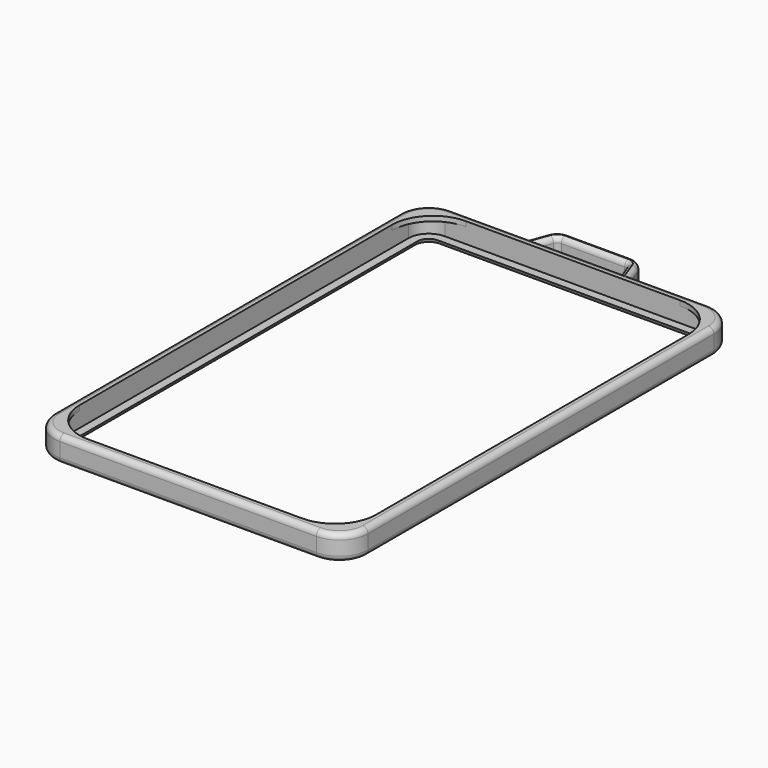
from build123d import *

# Parameters (mm, degrees)
F2_DEPTH      = 2.8
F4_DEPTH      = 0.9
F6_DEPTH      = 0.9
F8_DEPTH      = 3.7
F8_DEPTH_BACK = 0.9
F9_T1_DEPTH   = 79.28
F9_T3_DEPTH   = 11.5995849236
F9_T5_DEPTH   = 47.03
F9_T10_DEPTH  = 4.9923257792
F9_T15_DEPTH  = 20.1838214056
F9_T20_DEPTH  = 20.1838214056
F9_T26_DEPTH  = 20.1838214056
F9_T31_DEPTH  = 20.1838214056
F9_T36_DEPTH  = 20.1838214056
F9_T42_DEPTH  = 20.1838214056
F9_T45_ANGLE  = 90
F9_T47_ANGLE  = 90
F9_T49_ANGLE  = 90
F9_T51_ANGLE  = 90
F9_T53_ANGLE  = 90
F9_T57_DEPTH  = 16.7204048612
F9_T62_DEPTH  = 16.7204048612
F9_T67_DEPTH  = 16.7204048612
F9_T72_DEPTH  = 16.7204048612
F9_T75_ANGLE  = 90
F9_T77_ANGLE  = 90
F9_T81_DEPTH  = 16.7204048612
F9_T86_DEPTH  = 16.7204048612
F9_T91_DEPTH  = 16.7204048612
F9_T96_DEPTH  = 16.7204048612
F9_T99_ANGLE  = 90
F9_T101_ANGLE = 90
F9_T103_ANGLE = 90
F9_T105_ANGLE = 90
F9_T107_ANGLE = 90
F9_T109_ANGLE = 70
F9_T111_ANGLE = 70
F9_T115_DEPTH = 4.9923257792
F9_T120_DEPTH = 4.9923257792
F9_T123_ANGLE = 70
F9_T125_ANGLE = 70
F9_T129_DEPTH = 5.574678154
F9_T134_DEPTH = 5.574678154
F9_T137_ANGLE = 70
F9_T139_ANGLE = 70
F9_T143_DEPTH = 5.574678154
F9_T148_DEPTH = 5.574678154
F9_T151_ANGLE = 70
F9_T153_ANGLE = 70
F9_T157_DEPTH = 4.9923257792
F9_T163_DEPTH = 20.1838214056
F9_T168_DEPTH = 4.9923257792
F9_T175_DEPTH = 20.1838214056
F9_T180_DEPTH = 4.9923257792
F9_T187_DEPTH = 20.1838214056
F9_T192_DEPTH = 4.9923257792
F9_T199_DEPTH = 20.1838214056
F9_T204_DEPTH = 4.9923257792
F9_T211_DEPTH = 16.7204048612
F9_T216_DEPTH = 5.574678154
F9_T223_DEPTH = 5.574678154
F9_T227_DEPTH = 16.7204048612
F9_T235_DEPTH = 16.7204048612
F9_T240_DEPTH = 5.574678154
F9_T247_DEPTH = 5.574678154
F9_T251_DEPTH = 16.7204048612


# Not quite as in the source:
# - a fillet or chamfer that OpenCascade refuses, or shapes differently, is made with other operations: its cross-section is extruded or revolved along the edge and cut away or added


with BuildPart() as f2:
    # F1 (on Top) → F2 (new body)
    with BuildSketch(Plane.XY):
        with BuildLine():
            Line((-28.8, 39.64), (-28.8, -39.64))
            ThreePointArc((-28.8, -39.64), (-27.2520593386, -43.3770593386), (-23.515, -44.925))
            Line((-23.515, -44.925), (23.515, -44.925))
            ThreePointArc((23.515, -44.925), (27.2520593386, -43.3770593386), (28.8, -39.64))
            Line((28.8, -39.64), (28.8, 39.64))
            ThreePointArc((28.8, 39.64), (27.2520593386, 43.3770593386), (23.515, 44.925))
            Line((23.515, 44.925), (-23.515, 44.925))
            ThreePointArc((-23.515, 44.925), (-27.2520593386, 43.3770593386), (-28.8, 39.64))
        make_face()
        with BuildLine():
            ThreePointArc((-23.515, -43.325), (-26.1206884887, -42.2456884887), (-27.2, -39.64))
            Line((-27.2, -39.64), (-27.2, 39.64))
            ThreePointArc((-27.2, 39.64), (-26.1206884887, 42.2456884887), (-23.515, 43.325))
            Line((-23.515, 43.325), (23.515, 43.325))
            ThreePointArc((23.515, 43.325), (26.1206884887, 42.2456884887), (27.2, 39.64))
            Line((27.2, 39.64), (27.2, -39.64))
            ThreePointArc((27.2, -39.64), (26.1206884887, -42.2456884887), (23.515, -43.325))
            Line((23.515, -43.325), (-23.515, -43.325))
        make_face(mode=Mode.SUBTRACT)
    extrude(amount=F2_DEPTH)

    # F3 (on face) → F4 (join)
    with BuildSketch(Plane(origin=(0, 0, 0), x_dir=(1, 0, 0), z_dir=(0, 0, -1))):
        with BuildLine():
            Line((28.8, -39.64), (28.8, 39.64))
            ThreePointArc((28.8, 39.64), (27.2520593386, 43.3770593386), (23.515, 44.925))
            Line((23.515, 44.925), (-23.515, 44.925))
            ThreePointArc((-23.515, 44.925), (-27.2520593386, 43.3770593386), (-28.8, 39.64))
            Line((-28.8, 39.64), (-28.8, -39.64))
            ThreePointArc((-28.8, -39.64), (-27.2520593386, -43.3770593386), (-23.515, -44.925))
            Line((-23.515, -44.925), (23.515, -44.925))
            ThreePointArc((23.515, -44.925), (27.2520593386, -43.3770593386), (28.8, -39.64))
        make_face()
        with BuildLine():
            Line((-23.515, 43.325), (23.515, 43.325))
            ThreePointArc((23.515, 43.325), (26.1206884887, 42.2456884887), (27.2, 39.64))
            Line((27.2, 39.64), (27.2, -39.64))
            ThreePointArc((27.2, -39.64), (26.1206884887, -42.2456884887), (23.515, -43.325))
            Line((23.515, -43.325), (-23.515, -43.325))
            ThreePointArc((-23.515, -43.325), (-26.1206884887, -42.2456884887), (-27.2, -39.64))
            Line((-27.2, -39.64), (-27.2, 39.64))
            ThreePointArc((-27.2, 39.64), (-26.1206884887, 42.2456884887), (-23.515, 43.325))
        make_face(mode=Mode.SUBTRACT)
        with BuildLine():
            ThreePointArc((27.2, 39.64), (26.1206884887, 42.2456884887), (23.515, 43.325))
            Line((23.515, 43.325), (-23.515, 43.325))
            ThreePointArc((-23.515, 43.325), (-26.1206884887, 42.2456884887), (-27.2, 39.64))
            Line((-27.2, 39.64), (-27.2, -39.64))
            ThreePointArc((-27.2, -39.64), (-26.1206884887, -42.2456884887), (-23.515, -43.325))
            Line((-23.515, -43.325), (23.515, -43.325))
            ThreePointArc((23.515, -43.325), (26.1206884887, -42.2456884887), (27.2, -39.64))
            Line((27.2, -39.64), (27.2, 39.64))
        make_face()
        with BuildLine():
            Line((-25.6, -39.64), (-25.6, 39.64))
            ThreePointArc((-25.6, 39.64), (-24.9893176388, 41.1143176388), (-23.515, 41.725))
            Line((-23.515, 41.725), (23.515, 41.725))
            ThreePointArc((23.515, 41.725), (24.9893176388, 41.1143176388), (25.6, 39.64))
            Line((25.6, 39.64), (25.6, -39.64))
            ThreePointArc((25.6, -39.64), (24.9893176388, -41.1143176388), (23.515, -41.725))
            Line((23.515, -41.725), (-23.515, -41.725))
            ThreePointArc((-23.515, -41.725), (-24.9893176388, -41.1143176388), (-25.6, -39.64))
        make_face(mode=Mode.SUBTRACT)
    extrude(amount=F4_DEPTH)

    # F5 (on face) → F6 (join)
    with BuildSketch(Plane.XY.offset(2.8)):
        with BuildLine():
            Line((-23.515, -44.925), (23.515, -44.925))
            ThreePointArc((23.515, -44.925), (27.2520593386, -43.3770593386), (28.8, -39.64))
            Line((28.8, -39.64), (28.8, 39.64))
            ThreePointArc((28.8, 39.64), (27.2520593386, 43.3770593386), (23.515, 44.925))
            Line((23.515, 44.925), (-23.515, 44.925))
            ThreePointArc((-23.515, 44.925), (-27.2520593386, 43.3770593386), (-28.8, 39.64))
            Line((-28.8, 39.64), (-28.8, -39.64))
            ThreePointArc((-28.8, -39.64), (-27.2520593386, -43.3770593386), (-23.515, -44.925))
        make_face()
        with BuildLine():
            Line((19.6522583002, 43.325), (23.515, 43.325))
            ThreePointArc((23.515, 43.325), (26.1206884887, 42.2456884887), (27.2, 39.64))
            Line((27.2, 39.64), (27.2, 35.7772583002))
            Line((27.2, 35.7772583002), (27.2, -35.7772583002))
            Line((27.2, -35.7772583002), (27.2, -39.64))
            ThreePointArc((27.2, -39.64), (26.1206884887, -42.2456884887), (23.515, -43.325))
            Line((23.515, -43.325), (19.6522583002, -43.325))
            Line((19.6522583002, -43.325), (-19.6522583002, -43.325))
            Line((-19.6522583002, -43.325), (-23.515, -43.325))
            ThreePointArc((-23.515, -43.325), (-26.1206884887, -42.2456884887), (-27.2, -39.64))
            Line((-27.2, -39.64), (-27.2, -35.7772583002))
            Line((-27.2, -35.7772583002), (-27.2, 35.7772583002))
            Line((-27.2, 35.7772583002), (-27.2, 39.64))
            ThreePointArc((-27.2, 39.64), (-26.1206884887, 42.2456884887), (-23.515, 43.325))
            Line((-23.515, 43.325), (-19.6522583002, 43.325))
            Line((-19.6522583002, 43.325), (19.6522583002, 43.325))
        make_face(mode=Mode.SUBTRACT)
        with BuildLine():
            ThreePointArc((-27.2, 35.7772583002), (-24.9893176388, 41.1143176388), (-19.6522583002, 43.325))
            Line((-19.6522583002, 43.325), (-23.515, 43.325))
            ThreePointArc((-23.515, 43.325), (-26.1206884887, 42.2456884887), (-27.2, 39.64))
            Line((-27.2, 39.64), (-27.2, 35.7772583002))
        make_face()
        with BuildLine():
            ThreePointArc((27.2, 39.64), (26.1206884887, 42.2456884887), (23.515, 43.325))
            Line((23.515, 43.325), (19.6522583002, 43.325))
            ThreePointArc((19.6522583002, 43.325), (24.9893176388, 41.1143176388), (27.2, 35.7772583002))
            Line((27.2, 35.7772583002), (27.2, 39.64))
        make_face()
        with BuildLine():
            Line((27.2, -39.64), (27.2, -35.7772583002))
            ThreePointArc((27.2, -35.7772583002), (24.9893176388, -41.1143176388), (19.6522583002, -43.325))
            Line((19.6522583002, -43.325), (23.515, -43.325))
            ThreePointArc((23.515, -43.325), (26.1206884887, -42.2456884887), (27.2, -39.64))
        make_face()
        with BuildLine():
            ThreePointArc((-19.6522583002, -43.325), (-24.9893176388, -41.1143176388), (-27.2, -35.7772583002))
            Line((-27.2, -35.7772583002), (-27.2, -39.64))
            ThreePointArc((-27.2, -39.64), (-26.1206884887, -42.2456884887), (-23.515, -43.325))
            Line((-23.515, -43.325), (-19.6522583002, -43.325))
        make_face()
    extrude(amount=F6_DEPTH)

    # F7 (on Top) → F8 (join, two sides)
    with BuildSketch(Plane.XY) as f8_sk:
        with BuildLine():
            Line((-9.2945951388, 44.925), (-7.5919107028, 44.925))
            Line((-7.5919107028, 44.925), (-6.7394850826, 47.2670201433))
            ThreePointArc((-6.7394850826, 47.2670201433), (-6.3733688981, 47.7441520443), (-5.7997924618, 47.925))
            Line((-5.7997924618, 47.925), (5.7997924618, 47.925))
            ThreePointArc((5.7997924618, 47.925), (6.3733688981, 47.7441520443), (6.7394850826, 47.2670201433))
            Line((6.7394850826, 47.2670201433), (7.5919107028, 44.925))
            Line((7.5919107028, 44.925), (9.2945951388, 44.925))
            Line((9.2945951388, 44.925), (8.2429932758, 47.8142523726))
            ThreePointArc((8.2429932758, 47.8142523726), (7.2910911963, 49.0547953152), (5.7997924618, 49.525))
            Line((5.7997924618, 49.525), (-5.7997924618, 49.525))
            ThreePointArc((-5.7997924618, 49.525), (-7.2910911963, 49.0547953152), (-8.2429932758, 47.8142523726))
            Line((-8.2429932758, 47.8142523726), (-9.2945951388, 44.925))
        make_face()
    extrude(amount=F8_DEPTH)
    extrude(f8_sk.sketch, amount=-F8_DEPTH_BACK)

    # F9: fillet of radius 1 on 25 edges, made by hand

    # F9_s2 → F9_t1 (cut)
    with BuildSketch(Plane.XZ.offset(-39.64)):
        with BuildLine():
            ThreePointArc((-28.8, 2.7), (-28.5071067812, 3.4071067812), (-27.8, 3.7))
            Line((-27.8, 3.7), (-27.8, 3.72))
            Line((-27.8, 3.72), (-28.82, 3.72))
            Line((-28.82, 3.72), (-28.82, 2.7))
            Line((-28.82, 2.7), (-28.8, 2.7))
        make_face()
        with BuildLine():
            ThreePointArc((-28.8, 0.1), (-28.5071067812, -0.6071067812), (-27.8, -0.9))
            Line((-27.8, -0.9), (-27.8, -0.92))
            Line((-27.8, -0.92), (-28.82, -0.92))
            Line((-28.82, -0.92), (-28.82, 0.1))
            Line((-28.82, 0.1), (-28.8, 0.1))
        make_face()
        with BuildLine():
            ThreePointArc((-26.5949874371, -0.9), (-25.9241670439, -0.6416198487), (-25.6, 0))
            Line((-25.6, 0), (-25.5801002513, -0.002))
            ThreePointArc((-25.5801002513, -0.002), (-25.58, -0.45), (-25.58, -0.9))
            Line((-25.58, -0.9), (-25.6, -0.92))
            Line((-25.6, -0.92), (-26.5949874371, -0.92))
            Line((-26.5949874371, -0.92), (-26.5949874371, -0.9))
        make_face()
        with BuildLine():
            ThreePointArc((27.8, 3.7), (28.5071067812, 3.4071067812), (28.8, 2.7))
            Line((28.8, 2.7), (28.82, 2.7))
            Line((28.82, 2.7), (28.82, 3.72))
            Line((28.82, 3.72), (27.8, 3.72))
            Line((27.8, 3.72), (27.8, 3.7))
        make_face()
        with BuildLine():
            ThreePointArc((27.8, -0.9), (28.5071067812, -0.6071067812), (28.8, 0.1))
            Line((28.8, 0.1), (28.82, 0.1))
            Line((28.82, 0.1), (28.82, -0.92))
            Line((28.82, -0.92), (27.8, -0.92))
            Line((27.8, -0.92), (27.8, -0.9))
        make_face()
        with BuildLine():
            ThreePointArc((26.5949874371, -0.9), (25.9241670439, -0.6416198487), (25.6, 0))
            Line((25.6, 0), (25.5801002513, -0.002))
            ThreePointArc((25.5801002513, -0.002), (25.58, -0.45), (25.58, -0.9))
            Line((25.58, -0.9), (25.6, -0.92))
            Line((25.6, -0.92), (26.5949874371, -0.92))
            Line((26.5949874371, -0.92), (26.5949874371, -0.9))
        make_face()
    extrude(amount=F9_T1_DEPTH, mode=Mode.SUBTRACT)

    # F9_s4 → F9_t3 (cut)
    with BuildSketch(Plane.YZ.offset(-5.7997924618)):
        with BuildLine():
            ThreePointArc((48.525, -0.9), (49.2321067812, -0.6071067812), (49.525, 0.1))
            Line((49.525, 0.1), (49.545, 0.1))
            Line((49.545, 0.1), (49.545, -0.92))
            Line((49.545, -0.92), (48.525, -0.92))
            Line((48.525, -0.92), (48.525, -0.9))
        make_face()
        with BuildLine():
            ThreePointArc((48.525, 3.7), (49.2321067812, 3.4071067812), (49.525, 2.7))
            Line((49.525, 2.7), (49.545, 2.7))
            Line((49.545, 2.7), (49.545, 3.72))
            Line((49.545, 3.72), (48.525, 3.72))
            Line((48.525, 3.72), (48.525, 3.7))
        make_face()
        with BuildLine():
            ThreePointArc((48.925, -0.9), (48.2178932188, -0.6071067812), (47.925, 0.1))
            Line((47.925, 0.1), (47.905, 0.1))
            Line((47.905, 0.1), (47.905, -0.92))
            Line((47.905, -0.92), (48.925, -0.92))
            Line((48.925, -0.92), (48.925, -0.9))
        make_face()
        with BuildLine():
            ThreePointArc((48.925, 3.7), (48.2178932188, 3.4071067812), (47.925, 2.7))
            Line((47.925, 2.7), (47.905, 2.7))
            Line((47.905, 2.7), (47.905, 3.72))
            Line((47.905, 3.72), (48.925, 3.72))
            Line((48.925, 3.72), (48.925, 3.7))
        make_face()
    extrude(amount=F9_T3_DEPTH, mode=Mode.SUBTRACT)

    # F9_s6 → F9_t5 (cut)
    with BuildSketch(Plane.YZ.offset(-23.515)):
        with BuildLine():
            ThreePointArc((-43.925, 3.7), (-44.6321067812, 3.4071067812), (-44.925, 2.7))
            Line((-44.925, 2.7), (-44.945, 2.7))
            Line((-44.945, 2.7), (-44.945, 3.72))
            Line((-44.945, 3.72), (-43.925, 3.72))
            Line((-43.925, 3.72), (-43.925, 3.7))
        make_face()
        with BuildLine():
            ThreePointArc((-43.925, -0.9), (-44.6321067812, -0.6071067812), (-44.925, 0.1))
            Line((-44.925, 0.1), (-44.945, 0.1))
            Line((-44.945, 0.1), (-44.945, -0.92))
            Line((-44.945, -0.92), (-43.925, -0.92))
            Line((-43.925, -0.92), (-43.925, -0.9))
        make_face()
        with BuildLine():
            ThreePointArc((-42.7199874371, -0.9), (-42.0491670439, -0.6416198487), (-41.725, 0))
            Line((-41.725, 0), (-41.7051002513, -0.002))
            ThreePointArc((-41.7051002513, -0.002), (-41.705, -0.45), (-41.705, -0.9))
            Line((-41.705, -0.9), (-41.725, -0.92))
            Line((-41.725, -0.92), (-42.7199874371, -0.92))
            Line((-42.7199874371, -0.92), (-42.7199874371, -0.9))
        make_face()
        with BuildLine():
            ThreePointArc((42.7199874371, -0.9), (42.0491670439, -0.6416198487), (41.725, 0))
            Line((41.725, 0), (41.7051002513, -0.002))
            ThreePointArc((41.7051002513, -0.002), (41.705, -0.45), (41.705, -0.9))
            Line((41.705, -0.9), (41.725, -0.92))
            Line((41.725, -0.92), (42.7199874371, -0.92))
            Line((42.7199874371, -0.92), (42.7199874371, -0.9))
        make_face()
    extrude(amount=F9_T5_DEPTH, mode=Mode.SUBTRACT)


with BuildPart() as f9_tool8:
    # F9_s9 → F9_t10 (new body)
    with BuildSketch(Plane(origin=(12.6954814761, 34.8805486848, 0), x_dir=(0, 0, 1), z_dir=(0.3420201433, 0.9396926208, 0))):
        with BuildLine():
            ThreePointArc((3.7, -23.499317404), (3.4071067812, -22.7922106228), (2.7, -22.499317404))
            Line((2.7, -22.499317404), (2.7, -22.479317404))
            Line((2.7, -22.479317404), (3.72, -22.479317404))
            Line((3.72, -22.479317404), (3.72, -23.499317404))
            Line((3.72, -23.499317404), (3.7, -23.499317404))
        make_face()
    extrude(amount=F9_T10_DEPTH)

    split(bisect_by=Plane.XZ.offset(-44.925), keep=Keep.BOTTOM)


with BuildPart() as f2_1:
    add(f2.part)

    # F9_t7: cut F9_tool8
    add(f9_tool8.part, mode=Mode.SUBTRACT)


with BuildPart() as f9_tool13:
    # F9_s14 → F9_t15 (new body)
    with BuildSketch(Plane.YZ.offset(-10.0919107028)):
        with BuildLine():
            ThreePointArc((43.925, -0.9), (44.6321067812, -0.6071067812), (44.925, 0.1))
            Line((44.925, 0.1), (44.945, 0.1))
            Line((44.945, 0.1), (44.945, -0.92))
            Line((44.945, -0.92), (43.925, -0.92))
            Line((43.925, -0.92), (43.925, -0.9))
        make_face()
    extrude(amount=F9_T15_DEPTH)

    split(bisect_by=Plane(origin=(-22.6459507305, 8.2424519926, 0), x_dir=(0, 0, 1), z_dir=(-0.9396926208, 0.3420201433, 0)), keep=Keep.TOP)


with BuildPart() as f2_2:
    add(f2_1.part)

    # F9_t12: cut F9_tool13
    add(f9_tool13.part, mode=Mode.SUBTRACT)


with BuildPart() as f9_tool18:
    # F9_s19 → F9_t20 (new body)
    with BuildSketch(Plane.YZ.offset(-10.0919107028)):
        with BuildLine():
            ThreePointArc((43.925, -0.9), (44.6321067812, -0.6071067812), (44.925, 0.1))
            Line((44.925, 0.1), (44.945, 0.1))
            Line((44.945, 0.1), (44.945, -0.92))
            Line((44.945, -0.92), (43.925, -0.92))
            Line((43.925, -0.92), (43.925, -0.9))
        make_face()
    extrude(amount=F9_T20_DEPTH)

    split(bisect_by=Plane(origin=(21.1424425373, 7.6952197632, 0), x_dir=(0, 0, 1), z_dir=(-0.9396926208, -0.3420201433, 0)), keep=Keep.TOP)

    split(bisect_by=Plane(origin=(-21.1424425373, 7.6952197632, 0), x_dir=(0, 0, 1), z_dir=(0.9396926208, -0.3420201433, 0)), keep=Keep.TOP)


with BuildPart() as f2_3:
    add(f2_2.part)

    # F9_t17: cut F9_tool18
    add(f9_tool18.part, mode=Mode.SUBTRACT)


with BuildPart() as f9_tool24:
    # F9_s25 → F9_t26 (new body)
    with BuildSketch(Plane.YZ.offset(-10.0919107028)):
        with BuildLine():
            ThreePointArc((43.925, -0.9), (44.6321067812, -0.6071067812), (44.925, 0.1))
            Line((44.925, 0.1), (44.945, 0.1))
            Line((44.945, 0.1), (44.945, -0.92))
            Line((44.945, -0.92), (43.925, -0.92))
            Line((43.925, -0.92), (43.925, -0.9))
        make_face()
    extrude(amount=F9_T26_DEPTH)

    split(bisect_by=Plane(origin=(22.6459507305, 8.2424519926, 0), x_dir=(0, 0, 1), z_dir=(0.9396926208, 0.3420201433, 0)), keep=Keep.TOP)


with BuildPart() as f2_4:
    add(f2_3.part)

    # F9_t23: cut F9_tool24
    add(f9_tool24.part, mode=Mode.SUBTRACT)


with BuildPart() as f9_tool29:
    # F9_s30 → F9_t31 (new body)
    with BuildSketch(Plane.YZ.offset(10.0919107028)):
        with BuildLine():
            ThreePointArc((43.925, 3.7), (44.6321067812, 3.4071067812), (44.925, 2.7))
            Line((44.925, 2.7), (44.945, 2.7))
            Line((44.945, 2.7), (44.945, 3.72))
            Line((44.945, 3.72), (43.925, 3.72))
            Line((43.925, 3.72), (43.925, 3.7))
        make_face()
    extrude(amount=-F9_T31_DEPTH)

    split(bisect_by=Plane(origin=(22.6459507305, 8.2424519926, 0), x_dir=(0, 0, 1), z_dir=(0.9396926208, 0.3420201433, 0)), keep=Keep.TOP)


with BuildPart() as f2_5:
    add(f2_4.part)

    # F9_t28: cut F9_tool29
    add(f9_tool29.part, mode=Mode.SUBTRACT)


with BuildPart() as f9_tool34:
    # F9_s35 → F9_t36 (new body)
    with BuildSketch(Plane.YZ.offset(10.0919107028)):
        with BuildLine():
            ThreePointArc((43.925, 3.7), (44.6321067812, 3.4071067812), (44.925, 2.7))
            Line((44.925, 2.7), (44.945, 2.7))
            Line((44.945, 2.7), (44.945, 3.72))
            Line((44.945, 3.72), (43.925, 3.72))
            Line((43.925, 3.72), (43.925, 3.7))
        make_face()
    extrude(amount=-F9_T36_DEPTH)

    split(bisect_by=Plane(origin=(21.1424425373, 7.6952197632, 0), x_dir=(0, 0, 1), z_dir=(-0.9396926208, -0.3420201433, 0)), keep=Keep.TOP)

    split(bisect_by=Plane(origin=(-21.1424425373, 7.6952197632, 0), x_dir=(0, 0, 1), z_dir=(0.9396926208, -0.3420201433, 0)), keep=Keep.TOP)


with BuildPart() as f2_6:
    add(f2_5.part)

    # F9_t33: cut F9_tool34
    add(f9_tool34.part, mode=Mode.SUBTRACT)


with BuildPart() as f9_tool40:
    # F9_s41 → F9_t42 (new body)
    with BuildSketch(Plane.YZ.offset(10.0919107028)):
        with BuildLine():
            ThreePointArc((43.925, 3.7), (44.6321067812, 3.4071067812), (44.925, 2.7))
            Line((44.925, 2.7), (44.945, 2.7))
            Line((44.945, 2.7), (44.945, 3.72))
            Line((44.945, 3.72), (43.925, 3.72))
            Line((43.925, 3.72), (43.925, 3.7))
        make_face()
    extrude(amount=-F9_T42_DEPTH)

    split(bisect_by=Plane(origin=(-22.6459507305, 8.2424519926, 0), x_dir=(0, 0, 1), z_dir=(-0.9396926208, 0.3420201433, 0)), keep=Keep.TOP)


with BuildPart() as f2_7:
    add(f2_6.part)

    # F9_t39: cut F9_tool40
    add(f9_tool40.part, mode=Mode.SUBTRACT)

    # F9_s44 → F9_t45 (revolve, cut)
    with BuildSketch(Plane.YZ.offset(-23.515)):
        with BuildLine():
            ThreePointArc((44.925, 2.7), (44.6321067812, 3.4071067812), (43.925, 3.7))
            Line((43.925, 3.7), (43.925, 3.72))
            Line((43.925, 3.72), (44.945, 3.72))
            Line((44.945, 3.72), (44.945, 2.7))
            Line((44.945, 2.7), (44.925, 2.7))
        make_face()
    revolve(axis=Axis((-23.515, 39.64, 3.7), (0, 0, 1)), revolution_arc=F9_T45_ANGLE, mode=Mode.SUBTRACT)

    # F9_s46 → F9_t47 (revolve, cut)
    with BuildSketch(Plane.XZ.offset(-39.64)):
        with BuildLine():
            ThreePointArc((-28.8, 0.1), (-28.5071067812, -0.6071067812), (-27.8, -0.9))
            Line((-27.8, -0.9), (-27.8, -0.92))
            Line((-27.8, -0.92), (-28.82, -0.92))
            Line((-28.82, -0.92), (-28.82, 0.1))
            Line((-28.82, 0.1), (-28.8, 0.1))
        make_face()
    revolve(axis=Axis((-23.515, 39.64, -0.9), (0, 0, -1)), revolution_arc=F9_T47_ANGLE, mode=Mode.SUBTRACT)

    # F9_s48 → F9_t49 (revolve, cut)
    with BuildSketch(Plane.XZ.offset(39.64)):
        with BuildLine():
            ThreePointArc((-27.8, 3.7), (-28.5071067812, 3.4071067812), (-28.8, 2.7))
            Line((-28.8, 2.7), (-28.82, 2.7))
            Line((-28.82, 2.7), (-28.82, 3.72))
            Line((-28.82, 3.72), (-27.8, 3.72))
            Line((-27.8, 3.72), (-27.8, 3.7))
        make_face()
    revolve(axis=Axis((-23.515, -39.64, 3.7), (0, 0, 1)), revolution_arc=F9_T49_ANGLE, mode=Mode.SUBTRACT)

    # F9_s50 → F9_t51 (revolve, cut)
    with BuildSketch(Plane.YZ.offset(23.515)):
        with BuildLine():
            ThreePointArc((-43.925, 3.7), (-44.6321067812, 3.4071067812), (-44.925, 2.7))
            Line((-44.925, 2.7), (-44.945, 2.7))
            Line((-44.945, 2.7), (-44.945, 3.72))
            Line((-44.945, 3.72), (-43.925, 3.72))
            Line((-43.925, 3.72), (-43.925, 3.7))
        make_face()
    revolve(axis=Axis((23.515, -39.64, 3.7), (0, 0, 1)), revolution_arc=F9_T51_ANGLE, mode=Mode.SUBTRACT)

    # F9_s52 → F9_t53 (revolve, cut)
    with BuildSketch(Plane.XZ.offset(-39.64)):
        with BuildLine():
            ThreePointArc((27.8, 3.7), (28.5071067812, 3.4071067812), (28.8, 2.7))
            Line((28.8, 2.7), (28.82, 2.7))
            Line((28.82, 2.7), (28.82, 3.72))
            Line((28.82, 3.72), (27.8, 3.72))
            Line((27.8, 3.72), (27.8, 3.7))
        make_face()
    revolve(axis=Axis((23.515, 39.64, 3.7), (0, 0, 1)), revolution_arc=F9_T53_ANGLE, mode=Mode.SUBTRACT)


with BuildPart() as f9_tool55:
    # F9_s56 → F9_t57 (new body)
    with BuildSketch(Plane.YZ.offset(23.515)):
        with BuildLine():
            ThreePointArc((43.925, 3.7), (44.6321067812, 3.4071067812), (44.925, 2.7))
            Line((44.925, 2.7), (44.945, 2.7))
            Line((44.945, 2.7), (44.945, 3.72))
            Line((44.945, 3.72), (43.925, 3.72))
            Line((43.925, 3.72), (43.925, 3.7))
        make_face()
    extrude(amount=-F9_T57_DEPTH)

    split(bisect_by=Plane(origin=(22.6459507305, 8.2424519926, 0), x_dir=(0, 0, 1), z_dir=(0.9396926208, 0.3420201433, 0)), keep=Keep.TOP)


with BuildPart() as f2_8:
    add(f2_7.part)

    # F9_t54: cut F9_tool55
    add(f9_tool55.part, mode=Mode.SUBTRACT)


with BuildPart() as f9_tool60:
    # F9_s61 → F9_t62 (new body)
    with BuildSketch(Plane.YZ.offset(23.515)):
        with BuildLine():
            ThreePointArc((43.925, 3.7), (44.6321067812, 3.4071067812), (44.925, 2.7))
            Line((44.925, 2.7), (44.945, 2.7))
            Line((44.945, 2.7), (44.945, 3.72))
            Line((44.945, 3.72), (43.925, 3.72))
            Line((43.925, 3.72), (43.925, 3.7))
        make_face()
    extrude(amount=-F9_T62_DEPTH)

    split(bisect_by=Plane(origin=(21.1424425373, 7.6952197632, 0), x_dir=(0, 0, 1), z_dir=(-0.9396926208, -0.3420201433, 0)), keep=Keep.TOP)


with BuildPart() as f2_9:
    add(f2_8.part)

    # F9_t59: cut F9_tool60
    add(f9_tool60.part, mode=Mode.SUBTRACT)


with BuildPart() as f9_tool65:
    # F9_s66 → F9_t67 (new body)
    with BuildSketch(Plane.YZ.offset(-6.7945951388)):
        with BuildLine():
            ThreePointArc((43.925, 3.7), (44.6321067812, 3.4071067812), (44.925, 2.7))
            Line((44.925, 2.7), (44.945, 2.7))
            Line((44.945, 2.7), (44.945, 3.72))
            Line((44.945, 3.72), (43.925, 3.72))
            Line((43.925, 3.72), (43.925, 3.7))
        make_face()
    extrude(amount=-F9_T67_DEPTH)

    split(bisect_by=Plane(origin=(-21.1424425373, 7.6952197632, 0), x_dir=(0, 0, 1), z_dir=(0.9396926208, -0.3420201433, 0)), keep=Keep.TOP)


with BuildPart() as f2_10:
    add(f2_9.part)

    # F9_t64: cut F9_tool65
    add(f9_tool65.part, mode=Mode.SUBTRACT)


with BuildPart() as f9_tool70:
    # F9_s71 → F9_t72 (new body)
    with BuildSketch(Plane.YZ.offset(-6.7945951388)):
        with BuildLine():
            ThreePointArc((43.925, 3.7), (44.6321067812, 3.4071067812), (44.925, 2.7))
            Line((44.925, 2.7), (44.945, 2.7))
            Line((44.945, 2.7), (44.945, 3.72))
            Line((44.945, 3.72), (43.925, 3.72))
            Line((43.925, 3.72), (43.925, 3.7))
        make_face()
    extrude(amount=-F9_T72_DEPTH)

    split(bisect_by=Plane(origin=(-22.6459507305, 8.2424519926, 0), x_dir=(0, 0, 1), z_dir=(-0.9396926208, 0.3420201433, 0)), keep=Keep.TOP)


with BuildPart() as f2_11:
    add(f2_10.part)

    # F9_t69: cut F9_tool70
    add(f9_tool70.part, mode=Mode.SUBTRACT)

    # F9_s74 → F9_t75 (revolve, cut)
    with BuildSketch(Plane.YZ.offset(-23.515)):
        with BuildLine():
            ThreePointArc((-44.925, 0.1), (-44.6321067812, -0.6071067812), (-43.925, -0.9))
            Line((-43.925, -0.9), (-43.925, -0.92))
            Line((-43.925, -0.92), (-44.945, -0.92))
            Line((-44.945, -0.92), (-44.945, 0.1))
            Line((-44.945, 0.1), (-44.925, 0.1))
        make_face()
    revolve(axis=Axis((-23.515, -39.64, -0.9), (0, 0, -1)), revolution_arc=F9_T75_ANGLE, mode=Mode.SUBTRACT)

    # F9_s76 → F9_t77 (revolve, cut)
    with BuildSketch(Plane.XZ.offset(39.64)):
        with BuildLine():
            ThreePointArc((27.8, -0.9), (28.5071067812, -0.6071067812), (28.8, 0.1))
            Line((28.8, 0.1), (28.82, 0.1))
            Line((28.82, 0.1), (28.82, -0.92))
            Line((28.82, -0.92), (27.8, -0.92))
            Line((27.8, -0.92), (27.8, -0.9))
        make_face()
    revolve(axis=Axis((23.515, -39.64, -0.9), (0, 0, -1)), revolution_arc=F9_T77_ANGLE, mode=Mode.SUBTRACT)


with BuildPart() as f9_tool79:
    # F9_s80 → F9_t81 (new body)
    with BuildSketch(Plane.YZ.offset(-23.515)):
        with BuildLine():
            ThreePointArc((43.925, -0.9), (44.6321067812, -0.6071067812), (44.925, 0.1))
            Line((44.925, 0.1), (44.945, 0.1))
            Line((44.945, 0.1), (44.945, -0.92))
            Line((44.945, -0.92), (43.925, -0.92))
            Line((43.925, -0.92), (43.925, -0.9))
        make_face()
    extrude(amount=F9_T81_DEPTH)

    split(bisect_by=Plane(origin=(-22.6459507305, 8.2424519926, 0), x_dir=(0, 0, 1), z_dir=(-0.9396926208, 0.3420201433, 0)), keep=Keep.TOP)


with BuildPart() as f2_12:
    add(f2_11.part)

    # F9_t78: cut F9_tool79
    add(f9_tool79.part, mode=Mode.SUBTRACT)


with BuildPart() as f9_tool84:
    # F9_s85 → F9_t86 (new body)
    with BuildSketch(Plane.YZ.offset(-23.515)):
        with BuildLine():
            ThreePointArc((43.925, -0.9), (44.6321067812, -0.6071067812), (44.925, 0.1))
            Line((44.925, 0.1), (44.945, 0.1))
            Line((44.945, 0.1), (44.945, -0.92))
            Line((44.945, -0.92), (43.925, -0.92))
            Line((43.925, -0.92), (43.925, -0.9))
        make_face()
    extrude(amount=F9_T86_DEPTH)

    split(bisect_by=Plane(origin=(-21.1424425373, 7.6952197632, 0), x_dir=(0, 0, 1), z_dir=(0.9396926208, -0.3420201433, 0)), keep=Keep.TOP)


with BuildPart() as f2_13:
    add(f2_12.part)

    # F9_t83: cut F9_tool84
    add(f9_tool84.part, mode=Mode.SUBTRACT)


with BuildPart() as f9_tool89:
    # F9_s90 → F9_t91 (new body)
    with BuildSketch(Plane.YZ.offset(6.7945951388)):
        with BuildLine():
            ThreePointArc((43.925, -0.9), (44.6321067812, -0.6071067812), (44.925, 0.1))
            Line((44.925, 0.1), (44.945, 0.1))
            Line((44.945, 0.1), (44.945, -0.92))
            Line((44.945, -0.92), (43.925, -0.92))
            Line((43.925, -0.92), (43.925, -0.9))
        make_face()
    extrude(amount=F9_T91_DEPTH)

    split(bisect_by=Plane(origin=(21.1424425373, 7.6952197632, 0), x_dir=(0, 0, 1), z_dir=(-0.9396926208, -0.3420201433, 0)), keep=Keep.TOP)


with BuildPart() as f2_14:
    add(f2_13.part)

    # F9_t88: cut F9_tool89
    add(f9_tool89.part, mode=Mode.SUBTRACT)


with BuildPart() as f9_tool94:
    # F9_s95 → F9_t96 (new body)
    with BuildSketch(Plane.YZ.offset(6.7945951388)):
        with BuildLine():
            ThreePointArc((43.925, -0.9), (44.6321067812, -0.6071067812), (44.925, 0.1))
            Line((44.925, 0.1), (44.945, 0.1))
            Line((44.945, 0.1), (44.945, -0.92))
            Line((44.945, -0.92), (43.925, -0.92))
            Line((43.925, -0.92), (43.925, -0.9))
        make_face()
    extrude(amount=F9_T96_DEPTH)

    split(bisect_by=Plane(origin=(22.6459507305, 8.2424519926, 0), x_dir=(0, 0, 1), z_dir=(0.9396926208, 0.3420201433, 0)), keep=Keep.TOP)


with BuildPart() as f2_15:
    add(f2_14.part)

    # F9_t93: cut F9_tool94
    add(f9_tool94.part, mode=Mode.SUBTRACT)

    # F9_s98 → F9_t99 (revolve, cut)
    with BuildSketch(Plane.YZ.offset(23.515)):
        with BuildLine():
            ThreePointArc((43.925, -0.9), (44.6321067812, -0.6071067812), (44.925, 0.1))
            Line((44.925, 0.1), (44.945, 0.1))
            Line((44.945, 0.1), (44.945, -0.92))
            Line((44.945, -0.92), (43.925, -0.92))
            Line((43.925, -0.92), (43.925, -0.9))
        make_face()
    revolve(axis=Axis((23.515, 39.64, -0.9), (0, 0, -1)), revolution_arc=F9_T99_ANGLE, mode=Mode.SUBTRACT)

    # F9_s100 → F9_t101 (revolve, cut)
    with BuildSketch(Plane.YZ.offset(-23.515)):
        with BuildLine():
            ThreePointArc((42.7199874371, -0.9), (42.0491670439, -0.6416198487), (41.725, 0))
            Line((41.725, 0), (41.7051002513, -0.002))
            ThreePointArc((41.7051002513, -0.002), (41.705, -0.45), (41.705, -0.9))
            Line((41.705, -0.9), (41.725, -0.92))
            Line((41.725, -0.92), (42.7199874371, -0.92))
            Line((42.7199874371, -0.92), (42.7199874371, -0.9))
        make_face()
    revolve(axis=Axis((-23.515, 39.64, -0.9), (0, 0, 1)), revolution_arc=F9_T101_ANGLE, mode=Mode.SUBTRACT)

    # F9_s102 → F9_t103 (revolve, cut)
    with BuildSketch(Plane.XZ.offset(39.64)):
        with BuildLine():
            ThreePointArc((-26.5949874371, -0.9), (-25.9241670439, -0.6416198487), (-25.6, 0))
            Line((-25.6, 0), (-25.5801002513, -0.002))
            ThreePointArc((-25.5801002513, -0.002), (-25.58, -0.45), (-25.58, -0.9))
            Line((-25.58, -0.9), (-25.6, -0.92))
            Line((-25.6, -0.92), (-26.5949874371, -0.92))
            Line((-26.5949874371, -0.92), (-26.5949874371, -0.9))
        make_face()
    revolve(axis=Axis((-23.515, -39.64, -0.9), (0, 0, 1)), revolution_arc=F9_T103_ANGLE, mode=Mode.SUBTRACT)

    # F9_s104 → F9_t105 (revolve, cut)
    with BuildSketch(Plane.YZ.offset(23.515)):
        with BuildLine():
            ThreePointArc((-42.7199874371, -0.9), (-42.0491670439, -0.6416198487), (-41.725, 0))
            Line((-41.725, 0), (-41.7051002513, -0.002))
            ThreePointArc((-41.7051002513, -0.002), (-41.705, -0.45), (-41.705, -0.9))
            Line((-41.705, -0.9), (-41.725, -0.92))
            Line((-41.725, -0.92), (-42.7199874371, -0.92))
            Line((-42.7199874371, -0.92), (-42.7199874371, -0.9))
        make_face()
    revolve(axis=Axis((23.515, -39.64, -0.9), (0, 0, 1)), revolution_arc=F9_T105_ANGLE, mode=Mode.SUBTRACT)

    # F9_s106 → F9_t107 (revolve, cut)
    with BuildSketch(Plane.XZ.offset(-39.64)):
        with BuildLine():
            ThreePointArc((26.5949874371, -0.9), (25.9241670439, -0.6416198487), (25.6, 0))
            Line((25.6, 0), (25.5801002513, -0.002))
            ThreePointArc((25.5801002513, -0.002), (25.58, -0.45), (25.58, -0.9))
            Line((25.58, -0.9), (25.6, -0.92))
            Line((25.6, -0.92), (26.5949874371, -0.92))
            Line((26.5949874371, -0.92), (26.5949874371, -0.9))
        make_face()
    revolve(axis=Axis((23.515, 39.64, -0.9), (0, 0, 1)), revolution_arc=F9_T107_ANGLE, mode=Mode.SUBTRACT)

    # F9_s108 → F9_t109 (revolve, cut)
    with BuildSketch(Plane(origin=(14.4029574547, 39.5718003801, 0), x_dir=(0, 0, 1), z_dir=(-0.3420201433, -0.9396926208, 0))):
        with BuildLine():
            ThreePointArc((-0.9, 23.499317404), (-0.6071067812, 22.7922106228), (0.1, 22.499317404))
            Line((0.1, 22.499317404), (0.1, 22.479317404))
            Line((0.1, 22.479317404), (-0.92, 22.479317404))
            Line((-0.92, 22.479317404), (-0.92, 23.499317404))
            Line((-0.92, 23.499317404), (-0.9, 23.499317404))
        make_face()
    revolve(axis=Axis((-5.7997924618, 46.925, -0.9), (0, 0, -1)), revolution_arc=F9_T109_ANGLE, mode=Mode.SUBTRACT)

    # F9_s110 → F9_t111 (revolve, cut)
    with BuildSketch(Plane.YZ.offset(5.7997924618)):
        with BuildLine():
            ThreePointArc((48.925, -0.9), (48.2178932188, -0.6071067812), (47.925, 0.1))
            Line((47.925, 0.1), (47.905, 0.1))
            Line((47.905, 0.1), (47.905, -0.92))
            Line((47.905, -0.92), (48.925, -0.92))
            Line((48.925, -0.92), (48.925, -0.9))
        make_face()
    revolve(axis=Axis((5.7997924618, 46.925, -0.9), (0, 0, -1)), revolution_arc=F9_T111_ANGLE, mode=Mode.SUBTRACT)


with BuildPart() as f9_tool113:
    # F9_s114 → F9_t115 (new body)
    with BuildSketch(Plane(origin=(-14.4029574547, 39.5718003801, 0), x_dir=(0, 0, 1), z_dir=(0.3420201433, -0.9396926208, 0))):
        with BuildLine():
            ThreePointArc((-0.9, -23.499317404), (-0.6071067812, -22.7922106228), (0.1, -22.499317404))
            Line((0.1, -22.499317404), (0.1, -22.479317404))
            Line((0.1, -22.479317404), (-0.92, -22.479317404))
            Line((-0.92, -22.479317404), (-0.92, -23.499317404))
            Line((-0.92, -23.499317404), (-0.9, -23.499317404))
        make_face()
    extrude(amount=F9_T115_DEPTH)

    split(bisect_by=Plane.XZ.offset(-44.925), keep=Keep.BOTTOM)


with BuildPart() as f2_16:
    add(f2_15.part)

    # F9_t112: cut F9_tool113
    add(f9_tool113.part, mode=Mode.SUBTRACT)


with BuildPart() as f9_tool118:
    # F9_s119 → F9_t120 (new body)
    with BuildSketch(Plane(origin=(12.6954814761, 34.8805486848, 0), x_dir=(0, 0, 1), z_dir=(0.3420201433, 0.9396926208, 0))):
        with BuildLine():
            ThreePointArc((-0.9, -23.499317404), (-0.6071067812, -22.7922106228), (0.1, -22.499317404))
            Line((0.1, -22.499317404), (0.1, -22.479317404))
            Line((0.1, -22.479317404), (-0.92, -22.479317404))
            Line((-0.92, -22.479317404), (-0.92, -23.499317404))
            Line((-0.92, -23.499317404), (-0.9, -23.499317404))
        make_face()
    extrude(amount=F9_T120_DEPTH)

    split(bisect_by=Plane.XZ.offset(-44.925), keep=Keep.BOTTOM)


with BuildPart() as f2_17:
    add(f2_16.part)

    # F9_t117: cut F9_tool118
    add(f9_tool118.part, mode=Mode.SUBTRACT)

    # F9_s122 → F9_t123 (revolve, cut)
    with BuildSketch(Plane(origin=(-14.4029574547, 39.5718003801, 0), x_dir=(0, 0, 1), z_dir=(0.3420201433, -0.9396926208, 0))):
        with BuildLine():
            ThreePointArc((3.7, -23.099317404), (3.4071067812, -23.8064241852), (2.7, -24.099317404))
            Line((2.7, -24.099317404), (2.7, -24.119317404))
            Line((2.7, -24.119317404), (3.72, -24.119317404))
            Line((3.72, -24.119317404), (3.72, -23.099317404))
            Line((3.72, -23.099317404), (3.7, -23.099317404))
        make_face()
    revolve(axis=Axis((5.7997924618, 46.925, 3.7), (0, 0, 1)), revolution_arc=F9_T123_ANGLE, mode=Mode.SUBTRACT)

    # F9_s124 → F9_t125 (revolve, cut)
    with BuildSketch(Plane.YZ.offset(-5.7997924618)):
        with BuildLine():
            ThreePointArc((48.525, 3.7), (49.2321067812, 3.4071067812), (49.525, 2.7))
            Line((49.525, 2.7), (49.545, 2.7))
            Line((49.545, 2.7), (49.545, 3.72))
            Line((49.545, 3.72), (48.525, 3.72))
            Line((48.525, 3.72), (48.525, 3.7))
        make_face()
    revolve(axis=Axis((-5.7997924618, 46.925, 3.7), (0, 0, 1)), revolution_arc=F9_T125_ANGLE, mode=Mode.SUBTRACT)


with BuildPart() as f9_tool127:
    # F9_s128 → F9_t129 (new body)
    with BuildSketch(Plane(origin=(14.4029574547, 39.5718003801, 0), x_dir=(0, 0, 1), z_dir=(-0.3420201433, -0.9396926208, 0))):
        with BuildLine():
            ThreePointArc((3.7, 23.099317404), (3.4071067812, 23.8064241852), (2.7, 24.099317404))
            Line((2.7, 24.099317404), (2.7, 24.119317404))
            Line((2.7, 24.119317404), (3.72, 24.119317404))
            Line((3.72, 24.119317404), (3.72, 23.099317404))
            Line((3.72, 23.099317404), (3.7, 23.099317404))
        make_face()
    extrude(amount=F9_T129_DEPTH)

    split(bisect_by=Plane.XZ.offset(-44.925), keep=Keep.BOTTOM)


with BuildPart() as f2_18:
    add(f2_17.part)

    # F9_t126: cut F9_tool127
    add(f9_tool127.part, mode=Mode.SUBTRACT)


with BuildPart() as f9_tool132:
    # F9_s133 → F9_t134 (new body)
    with BuildSketch(Plane(origin=(-12.4963052334, 34.3333164555, 0), x_dir=(0, 0, 1), z_dir=(-0.3420201433, 0.9396926208, 0))):
        with BuildLine():
            ThreePointArc((3.7, 23.099317404), (3.4071067812, 23.8064241852), (2.7, 24.099317404))
            Line((2.7, 24.099317404), (2.7, 24.119317404))
            Line((2.7, 24.119317404), (3.72, 24.119317404))
            Line((3.72, 24.119317404), (3.72, 23.099317404))
            Line((3.72, 23.099317404), (3.7, 23.099317404))
        make_face()
    extrude(amount=F9_T134_DEPTH)

    split(bisect_by=Plane.XZ.offset(-44.925), keep=Keep.BOTTOM)


with BuildPart() as f2_19:
    add(f2_18.part)

    # F9_t131: cut F9_tool132
    add(f9_tool132.part, mode=Mode.SUBTRACT)

    # F9_s136 → F9_t137 (revolve, cut)
    with BuildSketch(Plane(origin=(-14.4029574547, 39.5718003801, 0), x_dir=(0, 0, 1), z_dir=(0.3420201433, -0.9396926208, 0))):
        with BuildLine():
            ThreePointArc((-0.9, -23.099317404), (-0.6071067812, -23.8064241852), (0.1, -24.099317404))
            Line((0.1, -24.099317404), (0.1, -24.119317404))
            Line((0.1, -24.119317404), (-0.92, -24.119317404))
            Line((-0.92, -24.119317404), (-0.92, -23.099317404))
            Line((-0.92, -23.099317404), (-0.9, -23.099317404))
        make_face()
    revolve(axis=Axis((5.7997924618, 46.925, -0.9), (0, 0, 1)), revolution_arc=F9_T137_ANGLE, mode=Mode.SUBTRACT)

    # F9_s138 → F9_t139 (revolve, cut)
    with BuildSketch(Plane.YZ.offset(-5.7997924618)):
        with BuildLine():
            ThreePointArc((48.525, -0.9), (49.2321067812, -0.6071067812), (49.525, 0.1))
            Line((49.525, 0.1), (49.545, 0.1))
            Line((49.545, 0.1), (49.545, -0.92))
            Line((49.545, -0.92), (48.525, -0.92))
            Line((48.525, -0.92), (48.525, -0.9))
        make_face()
    revolve(axis=Axis((-5.7997924618, 46.925, -0.9), (0, 0, 1)), revolution_arc=F9_T139_ANGLE, mode=Mode.SUBTRACT)


with BuildPart() as f9_tool141:
    # F9_s142 → F9_t143 (new body)
    with BuildSketch(Plane(origin=(14.4029574547, 39.5718003801, 0), x_dir=(0, 0, 1), z_dir=(-0.3420201433, -0.9396926208, 0))):
        with BuildLine():
            ThreePointArc((-0.9, 23.099317404), (-0.6071067812, 23.8064241852), (0.1, 24.099317404))
            Line((0.1, 24.099317404), (0.1, 24.119317404))
            Line((0.1, 24.119317404), (-0.92, 24.119317404))
            Line((-0.92, 24.119317404), (-0.92, 23.099317404))
            Line((-0.92, 23.099317404), (-0.9, 23.099317404))
        make_face()
    extrude(amount=F9_T143_DEPTH)

    split(bisect_by=Plane.XZ.offset(-44.925), keep=Keep.BOTTOM)


with BuildPart() as f2_20:
    add(f2_19.part)

    # F9_t140: cut F9_tool141
    add(f9_tool141.part, mode=Mode.SUBTRACT)


with BuildPart() as f9_tool146:
    # F9_s147 → F9_t148 (new body)
    with BuildSketch(Plane(origin=(-12.4963052334, 34.3333164555, 0), x_dir=(0, 0, 1), z_dir=(-0.3420201433, 0.9396926208, 0))):
        with BuildLine():
            ThreePointArc((-0.9, 23.099317404), (-0.6071067812, 23.8064241852), (0.1, 24.099317404))
            Line((0.1, 24.099317404), (0.1, 24.119317404))
            Line((0.1, 24.119317404), (-0.92, 24.119317404))
            Line((-0.92, 24.119317404), (-0.92, 23.099317404))
            Line((-0.92, 23.099317404), (-0.9, 23.099317404))
        make_face()
    extrude(amount=F9_T148_DEPTH)

    split(bisect_by=Plane.XZ.offset(-44.925), keep=Keep.BOTTOM)


with BuildPart() as f2_21:
    add(f2_20.part)

    # F9_t145: cut F9_tool146
    add(f9_tool146.part, mode=Mode.SUBTRACT)

    # F9_s150 → F9_t151 (revolve, cut)
    with BuildSketch(Plane(origin=(14.4029574547, 39.5718003801, 0), x_dir=(0, 0, 1), z_dir=(-0.3420201433, -0.9396926208, 0))):
        with BuildLine():
            ThreePointArc((3.7, 23.499317404), (3.4071067812, 22.7922106228), (2.7, 22.499317404))
            Line((2.7, 22.499317404), (2.7, 22.479317404))
            Line((2.7, 22.479317404), (3.72, 22.479317404))
            Line((3.72, 22.479317404), (3.72, 23.499317404))
            Line((3.72, 23.499317404), (3.7, 23.499317404))
        make_face()
    revolve(axis=Axis((-5.7997924618, 46.925, 3.7), (0, 0, -1)), revolution_arc=F9_T151_ANGLE, mode=Mode.SUBTRACT)

    # F9_s152 → F9_t153 (revolve, cut)
    with BuildSketch(Plane.YZ.offset(5.7997924618)):
        with BuildLine():
            ThreePointArc((48.925, 3.7), (48.2178932188, 3.4071067812), (47.925, 2.7))
            Line((47.925, 2.7), (47.905, 2.7))
            Line((47.905, 2.7), (47.905, 3.72))
            Line((47.905, 3.72), (48.925, 3.72))
            Line((48.925, 3.72), (48.925, 3.7))
        make_face()
    revolve(axis=Axis((5.7997924618, 46.925, 3.7), (0, 0, -1)), revolution_arc=F9_T153_ANGLE, mode=Mode.SUBTRACT)


with BuildPart() as f9_tool155:
    # F9_s156 → F9_t157 (new body)
    with BuildSketch(Plane(origin=(-14.4029574547, 39.5718003801, 0), x_dir=(0, 0, 1), z_dir=(0.3420201433, -0.9396926208, 0))):
        with BuildLine():
            ThreePointArc((3.7, -23.499317404), (3.4071067812, -22.7922106228), (2.7, -22.499317404))
            Line((2.7, -22.499317404), (2.7, -22.479317404))
            Line((2.7, -22.479317404), (3.72, -22.479317404))
            Line((3.72, -22.479317404), (3.72, -23.499317404))
            Line((3.72, -23.499317404), (3.7, -23.499317404))
        make_face()
    extrude(amount=F9_T157_DEPTH)

    split(bisect_by=Plane.XZ.offset(-44.925), keep=Keep.BOTTOM)


with BuildPart() as f2_22:
    add(f2_21.part)

    # F9_t154: cut F9_tool155
    add(f9_tool155.part, mode=Mode.SUBTRACT)


with BuildPart() as f9_tool161:
    # F9_s162 → F9_t163 (new body)
    with BuildSketch(Plane.YZ.offset(10.0919107028)):
        with BuildLine():
            ThreePointArc((43.925, 3.7), (44.6321067812, 3.4071067812), (44.925, 2.7))
            Line((44.925, 2.7), (44.945, 2.7))
            Line((44.945, 2.7), (44.945, 3.72))
            Line((44.945, 3.72), (43.925, 3.72))
            Line((43.925, 3.72), (43.925, 3.7))
        make_face()
    extrude(amount=-F9_T163_DEPTH)

    split(bisect_by=Plane(origin=(-22.6459507305, 8.2424519926, 0), x_dir=(0, 0, 1), z_dir=(0.9396926208, -0.3420201433, 0)), keep=Keep.TOP)

    split(bisect_by=Plane(origin=(-21.1424425373, 7.6952197632, 0), x_dir=(0, 0, 1), z_dir=(-0.9396926208, 0.3420201433, 0)), keep=Keep.TOP)


with BuildPart() as f9_tool166:
    # F9_s167 → F9_t168 (new body)
    with BuildSketch(Plane(origin=(12.6954814761, 34.8805486848, 0), x_dir=(0, 0, 1), z_dir=(0.3420201433, 0.9396926208, 0))):
        with BuildLine():
            ThreePointArc((3.7, -23.499317404), (3.4071067812, -22.7922106228), (2.7, -22.499317404))
            Line((2.7, -22.499317404), (2.7, -22.479317404))
            Line((2.7, -22.479317404), (3.72, -22.479317404))
            Line((3.72, -22.479317404), (3.72, -23.499317404))
            Line((3.72, -23.499317404), (3.7, -23.499317404))
        make_face()
    extrude(amount=F9_T168_DEPTH)

    split(bisect_by=Plane.XZ.offset(-44.925), keep=Keep.TOP)


with BuildPart() as f9_tool161_1:
    add(f9_tool161.part)

    # F9_t170: intersect F9_tool166
    add(f9_tool166.part, mode=Mode.INTERSECT)


with BuildPart() as f2_23:
    add(f2_22.part)

    # F9_t159: cut F9_tool161
    add(f9_tool161_1.part, mode=Mode.SUBTRACT)


with BuildPart() as f9_tool173:
    # F9_s174 → F9_t175 (new body)
    with BuildSketch(Plane.YZ.offset(-10.0919107028)):
        with BuildLine():
            ThreePointArc((43.925, -0.9), (44.6321067812, -0.6071067812), (44.925, 0.1))
            Line((44.925, 0.1), (44.945, 0.1))
            Line((44.945, 0.1), (44.945, -0.92))
            Line((44.945, -0.92), (43.925, -0.92))
            Line((43.925, -0.92), (43.925, -0.9))
        make_face()
    extrude(amount=F9_T175_DEPTH)

    split(bisect_by=Plane(origin=(-22.6459507305, 8.2424519926, 0), x_dir=(0, 0, 1), z_dir=(0.9396926208, -0.3420201433, 0)), keep=Keep.TOP)

    split(bisect_by=Plane(origin=(-21.1424425373, 7.6952197632, 0), x_dir=(0, 0, 1), z_dir=(-0.9396926208, 0.3420201433, 0)), keep=Keep.TOP)


with BuildPart() as f9_tool178:
    # F9_s179 → F9_t180 (new body)
    with BuildSketch(Plane(origin=(12.6954814761, 34.8805486848, 0), x_dir=(0, 0, 1), z_dir=(0.3420201433, 0.9396926208, 0))):
        with BuildLine():
            ThreePointArc((-0.9, -23.499317404), (-0.6071067812, -22.7922106228), (0.1, -22.499317404))
            Line((0.1, -22.499317404), (0.1, -22.479317404))
            Line((0.1, -22.479317404), (-0.92, -22.479317404))
            Line((-0.92, -22.479317404), (-0.92, -23.499317404))
            Line((-0.92, -23.499317404), (-0.9, -23.499317404))
        make_face()
    extrude(amount=F9_T180_DEPTH)

    split(bisect_by=Plane.XZ.offset(-44.925), keep=Keep.TOP)


with BuildPart() as f9_tool173_1:
    add(f9_tool173.part)

    # F9_t182: intersect F9_tool178
    add(f9_tool178.part, mode=Mode.INTERSECT)


with BuildPart() as f2_24:
    add(f2_23.part)

    # F9_t171: cut F9_tool173
    add(f9_tool173_1.part, mode=Mode.SUBTRACT)


with BuildPart() as f9_tool185:
    # F9_s186 → F9_t187 (new body)
    with BuildSketch(Plane.YZ.offset(-10.0919107028)):
        with BuildLine():
            ThreePointArc((43.925, -0.9), (44.6321067812, -0.6071067812), (44.925, 0.1))
            Line((44.925, 0.1), (44.945, 0.1))
            Line((44.945, 0.1), (44.945, -0.92))
            Line((44.945, -0.92), (43.925, -0.92))
            Line((43.925, -0.92), (43.925, -0.9))
        make_face()
    extrude(amount=F9_T187_DEPTH)

    split(bisect_by=Plane(origin=(22.6459507305, 8.2424519926, 0), x_dir=(0, 0, 1), z_dir=(-0.9396926208, -0.3420201433, 0)), keep=Keep.TOP)

    split(bisect_by=Plane(origin=(21.1424425373, 7.6952197632, 0), x_dir=(0, 0, 1), z_dir=(0.9396926208, 0.3420201433, 0)), keep=Keep.TOP)


with BuildPart() as f9_tool190:
    # F9_s191 → F9_t192 (new body)
    with BuildSketch(Plane(origin=(-14.4029574547, 39.5718003801, 0), x_dir=(0, 0, 1), z_dir=(0.3420201433, -0.9396926208, 0))):
        with BuildLine():
            ThreePointArc((-0.9, -23.499317404), (-0.6071067812, -22.7922106228), (0.1, -22.499317404))
            Line((0.1, -22.499317404), (0.1, -22.479317404))
            Line((0.1, -22.479317404), (-0.92, -22.479317404))
            Line((-0.92, -22.479317404), (-0.92, -23.499317404))
            Line((-0.92, -23.499317404), (-0.9, -23.499317404))
        make_face()
    extrude(amount=F9_T192_DEPTH)

    split(bisect_by=Plane.XZ.offset(-44.925), keep=Keep.TOP)


with BuildPart() as f9_tool185_1:
    add(f9_tool185.part)

    # F9_t194: intersect F9_tool190
    add(f9_tool190.part, mode=Mode.INTERSECT)


with BuildPart() as f2_25:
    add(f2_24.part)

    # F9_t183: cut F9_tool185
    add(f9_tool185_1.part, mode=Mode.SUBTRACT)


with BuildPart() as f9_tool197:
    # F9_s198 → F9_t199 (new body)
    with BuildSketch(Plane.YZ.offset(10.0919107028)):
        with BuildLine():
            ThreePointArc((43.925, 3.7), (44.6321067812, 3.4071067812), (44.925, 2.7))
            Line((44.925, 2.7), (44.945, 2.7))
            Line((44.945, 2.7), (44.945, 3.72))
            Line((44.945, 3.72), (43.925, 3.72))
            Line((43.925, 3.72), (43.925, 3.7))
        make_face()
    extrude(amount=-F9_T199_DEPTH)

    split(bisect_by=Plane(origin=(22.6459507305, 8.2424519926, 0), x_dir=(0, 0, 1), z_dir=(-0.9396926208, -0.3420201433, 0)), keep=Keep.TOP)

    split(bisect_by=Plane(origin=(21.1424425373, 7.6952197632, 0), x_dir=(0, 0, 1), z_dir=(0.9396926208, 0.3420201433, 0)), keep=Keep.TOP)


with BuildPart() as f9_tool202:
    # F9_s203 → F9_t204 (new body)
    with BuildSketch(Plane(origin=(-14.4029574547, 39.5718003801, 0), x_dir=(0, 0, 1), z_dir=(0.3420201433, -0.9396926208, 0))):
        with BuildLine():
            ThreePointArc((3.7, -23.499317404), (3.4071067812, -22.7922106228), (2.7, -22.499317404))
            Line((2.7, -22.499317404), (2.7, -22.479317404))
            Line((2.7, -22.479317404), (3.72, -22.479317404))
            Line((3.72, -22.479317404), (3.72, -23.499317404))
            Line((3.72, -23.499317404), (3.7, -23.499317404))
        make_face()
    extrude(amount=F9_T204_DEPTH)

    split(bisect_by=Plane.XZ.offset(-44.925), keep=Keep.TOP)


with BuildPart() as f9_tool197_1:
    add(f9_tool197.part)

    # F9_t206: intersect F9_tool202
    add(f9_tool202.part, mode=Mode.INTERSECT)


with BuildPart() as f2_26:
    add(f2_25.part)

    # F9_t195: cut F9_tool197
    add(f9_tool197_1.part, mode=Mode.SUBTRACT)


with BuildPart() as f9_tool209:
    # F9_s210 → F9_t211 (new body)
    with BuildSketch(Plane.YZ.offset(23.515)):
        with BuildLine():
            ThreePointArc((43.925, 3.7), (44.6321067812, 3.4071067812), (44.925, 2.7))
            Line((44.925, 2.7), (44.945, 2.7))
            Line((44.945, 2.7), (44.945, 3.72))
            Line((44.945, 3.72), (43.925, 3.72))
            Line((43.925, 3.72), (43.925, 3.7))
        make_face()
    extrude(amount=-F9_T211_DEPTH)

    split(bisect_by=Plane(origin=(22.6459507305, 8.2424519926, 0), x_dir=(0, 0, 1), z_dir=(-0.9396926208, -0.3420201433, 0)), keep=Keep.TOP)

    split(bisect_by=Plane(origin=(21.1424425373, 7.6952197632, 0), x_dir=(0, 0, 1), z_dir=(0.9396926208, 0.3420201433, 0)), keep=Keep.TOP)


with BuildPart() as f9_tool214:
    # F9_s215 → F9_t216 (new body)
    with BuildSketch(Plane(origin=(-12.4963052334, 34.3333164555, 0), x_dir=(0, 0, 1), z_dir=(-0.3420201433, 0.9396926208, 0))):
        with BuildLine():
            ThreePointArc((3.7, 23.099317404), (3.4071067812, 23.8064241852), (2.7, 24.099317404))
            Line((2.7, 24.099317404), (2.7, 24.119317404))
            Line((2.7, 24.119317404), (3.72, 24.119317404))
            Line((3.72, 24.119317404), (3.72, 23.099317404))
            Line((3.72, 23.099317404), (3.7, 23.099317404))
        make_face()
    extrude(amount=F9_T216_DEPTH)

    split(bisect_by=Plane.XZ.offset(-44.925), keep=Keep.TOP)


with BuildPart() as f9_tool209_1:
    add(f9_tool209.part)

    # F9_t218: intersect F9_tool214
    add(f9_tool214.part, mode=Mode.INTERSECT)


with BuildPart() as f2_27:
    add(f2_26.part)

    # F9_t207: cut F9_tool209
    add(f9_tool209_1.part, mode=Mode.SUBTRACT)


with BuildPart() as f9_tool221:
    # F9_s222 → F9_t223 (new body)
    with BuildSketch(Plane(origin=(14.4029574547, 39.5718003801, 0), x_dir=(0, 0, 1), z_dir=(-0.3420201433, -0.9396926208, 0))):
        with BuildLine():
            ThreePointArc((3.7, 23.099317404), (3.4071067812, 23.8064241852), (2.7, 24.099317404))
            Line((2.7, 24.099317404), (2.7, 24.119317404))
            Line((2.7, 24.119317404), (3.72, 24.119317404))
            Line((3.72, 24.119317404), (3.72, 23.099317404))
            Line((3.72, 23.099317404), (3.7, 23.099317404))
        make_face()
    extrude(amount=F9_T223_DEPTH)

    split(bisect_by=Plane.XZ.offset(-44.925), keep=Keep.TOP)


with BuildPart() as f9_tool225:
    # F9_s226 → F9_t227 (new body)
    with BuildSketch(Plane.YZ.offset(-6.7945951388)):
        with BuildLine():
            ThreePointArc((43.925, 3.7), (44.6321067812, 3.4071067812), (44.925, 2.7))
            Line((44.925, 2.7), (44.945, 2.7))
            Line((44.945, 2.7), (44.945, 3.72))
            Line((44.945, 3.72), (43.925, 3.72))
            Line((43.925, 3.72), (43.925, 3.7))
        make_face()
    extrude(amount=-F9_T227_DEPTH)

    split(bisect_by=Plane(origin=(-22.6459507305, 8.2424519926, 0), x_dir=(0, 0, 1), z_dir=(0.9396926208, -0.3420201433, 0)), keep=Keep.TOP)

    split(bisect_by=Plane(origin=(-21.1424425373, 7.6952197632, 0), x_dir=(0, 0, 1), z_dir=(-0.9396926208, 0.3420201433, 0)), keep=Keep.TOP)


with BuildPart() as f9_tool221_1:
    add(f9_tool221.part)

    # F9_t230: intersect F9_tool225
    add(f9_tool225.part, mode=Mode.INTERSECT)


with BuildPart() as f2_28:
    add(f2_27.part)

    # F9_t219: cut F9_tool221
    add(f9_tool221_1.part, mode=Mode.SUBTRACT)


with BuildPart() as f9_tool233:
    # F9_s234 → F9_t235 (new body)
    with BuildSketch(Plane.YZ.offset(-23.515)):
        with BuildLine():
            ThreePointArc((43.925, -0.9), (44.6321067812, -0.6071067812), (44.925, 0.1))
            Line((44.925, 0.1), (44.945, 0.1))
            Line((44.945, 0.1), (44.945, -0.92))
            Line((44.945, -0.92), (43.925, -0.92))
            Line((43.925, -0.92), (43.925, -0.9))
        make_face()
    extrude(amount=F9_T235_DEPTH)

    split(bisect_by=Plane(origin=(-22.6459507305, 8.2424519926, 0), x_dir=(0, 0, 1), z_dir=(0.9396926208, -0.3420201433, 0)), keep=Keep.TOP)

    split(bisect_by=Plane(origin=(-21.1424425373, 7.6952197632, 0), x_dir=(0, 0, 1), z_dir=(-0.9396926208, 0.3420201433, 0)), keep=Keep.TOP)


with BuildPart() as f9_tool238:
    # F9_s239 → F9_t240 (new body)
    with BuildSketch(Plane(origin=(14.4029574547, 39.5718003801, 0), x_dir=(0, 0, 1), z_dir=(-0.3420201433, -0.9396926208, 0))):
        with BuildLine():
            ThreePointArc((-0.9, 23.099317404), (-0.6071067812, 23.8064241852), (0.1, 24.099317404))
            Line((0.1, 24.099317404), (0.1, 24.119317404))
            Line((0.1, 24.119317404), (-0.92, 24.119317404))
            Line((-0.92, 24.119317404), (-0.92, 23.099317404))
            Line((-0.92, 23.099317404), (-0.9, 23.099317404))
        make_face()
    extrude(amount=F9_T240_DEPTH)

    split(bisect_by=Plane.XZ.offset(-44.925), keep=Keep.TOP)


with BuildPart() as f9_tool233_1:
    add(f9_tool233.part)

    # F9_t242: intersect F9_tool238
    add(f9_tool238.part, mode=Mode.INTERSECT)


with BuildPart() as f2_29:
    add(f2_28.part)

    # F9_t231: cut F9_tool233
    add(f9_tool233_1.part, mode=Mode.SUBTRACT)


with BuildPart() as f9_tool245:
    # F9_s246 → F9_t247 (new body)
    with BuildSketch(Plane(origin=(-12.4963052334, 34.3333164555, 0), x_dir=(0, 0, 1), z_dir=(-0.3420201433, 0.9396926208, 0))):
        with BuildLine():
            ThreePointArc((-0.9, 23.099317404), (-0.6071067812, 23.8064241852), (0.1, 24.099317404))
            Line((0.1, 24.099317404), (0.1, 24.119317404))
            Line((0.1, 24.119317404), (-0.92, 24.119317404))
            Line((-0.92, 24.119317404), (-0.92, 23.099317404))
            Line((-0.92, 23.099317404), (-0.9, 23.099317404))
        make_face()
    extrude(amount=F9_T247_DEPTH)

    split(bisect_by=Plane.XZ.offset(-44.925), keep=Keep.TOP)


with BuildPart() as f9_tool249:
    # F9_s250 → F9_t251 (new body)
    with BuildSketch(Plane.YZ.offset(6.7945951388)):
        with BuildLine():
            ThreePointArc((43.925, -0.9), (44.6321067812, -0.6071067812), (44.925, 0.1))
            Line((44.925, 0.1), (44.945, 0.1))
            Line((44.945, 0.1), (44.945, -0.92))
            Line((44.945, -0.92), (43.925, -0.92))
            Line((43.925, -0.92), (43.925, -0.9))
        make_face()
    extrude(amount=F9_T251_DEPTH)

    split(bisect_by=Plane(origin=(22.6459507305, 8.2424519926, 0), x_dir=(0, 0, 1), z_dir=(-0.9396926208, -0.3420201433, 0)), keep=Keep.TOP)

    split(bisect_by=Plane(origin=(21.1424425373, 7.6952197632, 0), x_dir=(0, 0, 1), z_dir=(0.9396926208, 0.3420201433, 0)), keep=Keep.TOP)


with BuildPart() as f9_tool245_1:
    add(f9_tool245.part)

    # F9_t254: intersect F9_tool249
    add(f9_tool249.part, mode=Mode.INTERSECT)


with BuildPart() as f2_30:
    add(f2_29.part)

    # F9_t243: cut F9_tool245
    add(f9_tool245_1.part, mode=Mode.SUBTRACT)


solid = f2_30.part
